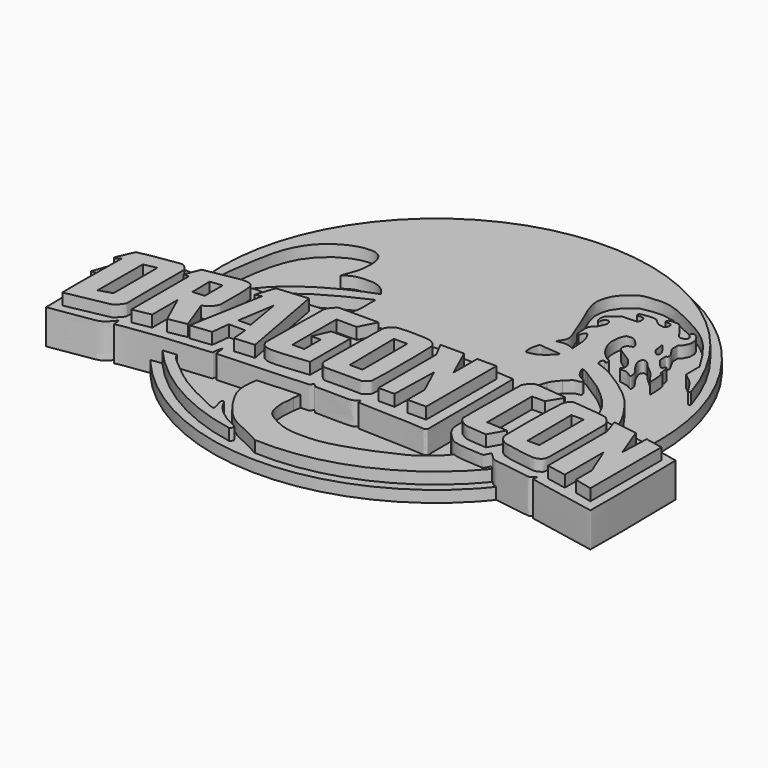
from build123d import *

# Parameters (mm, degrees)
F4_DEPTH = 6
F5_DEPTH = 9
F6_DEPTH = 12
F3_R     = 58.2680321176
F3_R_2   = 56.2680321176
F7_DEPTH = 3


with BuildPart() as f4:
    # F0 (on Top) → F4 (new body)
    with BuildSketch(Plane.XY):
        with BuildLine():
            ThreePointArc((50.2046270682, 32.5990865515), (-16.7313832275, 70.5566357957), (-58.0834932625, 5.662814714))
            add(Edge.make_bspline(
                [(-56.7946247756, 5.2932645194), (-56.9072491765, 5.3525443032), (-57.1453488244, 5.4763741354), (-57.5821193773, 5.672389242), (-57.9185015008, 5.6612390893), (-58.0834932625, 5.662814714)],
                knots=[0, 0, 0, 0, 0.3106893035, 0.6504797755, 1, 1, 1, 1], degree=3))
            add(Edge.make_bspline(
                [(-56.7946247756, 5.634940695), (-56.7946247756, 5.5210486365), (-56.7946247756, 5.407156578), (-56.7946247756, 5.2932645194)],
                knots=[0, 0, 0, 0, 0.3416761756, 0.3416761756, 0.3416761756, 0.3416761756], degree=3))
            add(Edge.make_bspline(
                [(-56.7946247756, 5.634940695), (-56.743940958, 7.2671798267), (-56.6456838315, 10.4314861922), (-56.7331520593, 14.5389266601), (-55.4633891473, 22.7353611724), (-54.1617687318, 29.6389256337), (-50.5897890483, 36.1168723343), (-44.7304711778, 39.9612863347), (-40.4860770295, 40.8741166974), (-37.6101297308, 40.5829749813), (-36.0593532544, 38.4827961794), (-35.7341565041, 35.7735493388), (-36.0278357089, 32.4009184257), (-36.969322235, 30.1083105362), (-37.420851473, 28.7852784917), (-37.6350395381, 28.1576830894)],
                knots=[0, 0, 0, 0, 0.0811415104, 0.1573032975, 0.2640365926, 0.3647803654, 0.4649779823, 0.5628837924, 0.6401346208, 0.7006202399, 0.7574588792, 0.8192083533, 0.8879467994, 0.946846281, 1, 1, 1, 1], degree=3))
            add(Edge.make_bspline(
                [(-37.6350395381, 28.1576830894), (-36.9020123713, 28.6742797134), (-35.3625484353, 29.7592079508), (-32.0226096017, 30.0311701045), (-28.9781587103, 29.8321241822), (-26.8192759482, 28.0309743743), (-26.3082476936, 27.1731155382), (-26.0944720358, 26.8142521381)],
                knots=[0, 0, 0, 0, 0.2057371384, 0.4320779901, 0.6506279419, 0.8538490957, 1, 1, 1, 1], degree=3))
            add(Edge.make_bspline(
                [(-50.9683191776, 7.4282060377), (-50.0897355561, 9.1461288779), (-48.1549941281, 12.9291910788), (-42.0082562909, 19.0156346462), (-32.7576914853, 24.3042127224), (-28.1550707663, 26.0380231586), (-26.0944720358, 26.8142521381)],
                knots=[0, 0, 0, 0, 0.2162082281, 0.4761151991, 0.7654561561, 1, 1, 1, 1], degree=3))
            add(Edge.make_bspline(
                [(-50.9683191776, 7.4282060377), (-50.5346785598, 7.504976032), (-49.5772579756, 7.674473929), (-48.2885622292, 7.7307833579), (-47.5835502148, 7.7615887858)],
                knots=[0, 0, 0, 0, 0.4529259397, 1, 1, 1, 1], degree=3))
            add(Edge.make_bspline(
                [(-25.3540985286, 24.1653900594), (-26.8552881088, 23.4932910546), (-30.1240573245, 22.0298273017), (-36.579939726, 18.4844991642), (-40.5144127202, 15.6900251466), (-44.4997206983, 12.1915121861), (-46.2658510708, 9.8325827108), (-47.1601372748, 8.4270560364), (-47.5835502148, 7.7615887858)],
                knots=[0, 0, 0, 0, 0.1794087162, 0.3906539828, 0.5668669146, 0.7447237719, 0.8791357199, 1, 1, 1, 1], degree=3))
            add(Edge.make_bspline(
                [(-27.7303513139, 12.6673979685), (-27.2486818484, 13.2179868784), (-26.3076778392, 14.2936339948), (-26.1352969689, 16.242044308), (-25.1319103155, 19.098439079), (-25.4017287693, 21.912956441), (-25.3693180923, 23.4456570399), (-25.3540985286, 24.1653900594)],
                knots=[0, 0, 0, 0, 0.186897327, 0.3651282604, 0.5890583856, 0.8070280333, 1, 1, 1, 1], degree=3))
            add(Edge.make_bspline(
                [(-27.7303513139, 12.6673979685), (-27.3267480987, 12.711642758), (-26.4365206138, 12.8092334765), (-24.8125175039, 11.887978411), (-23.3858019743, 10.910104507), (-22.5945804268, 10.3677995503)],
                knots=[0, 0, 0, 0, 0.2697704197, 0.5950325299, 1, 1, 1, 1], degree=3))
            add(Edge.make_bspline(
                [(-22.5945804268, 10.3677995503), (-22.4494425383, 10.1692900968), (-22.1047770931, 9.6978808054), (-20.541269939, 10.4450566992), (12.4683706928, 10.6003936274), (19.1899524017, 10.0772365955), (21.6048229486, 9.8892813548)],
                knots=[0, 0, 0, 0, 0.0748352198, 0.1777145488, 0.7045765412, 1, 1, 1, 1], degree=3))
            add(Edge.make_bspline(
                [(22.3375074565, 6.7731132731), (22.2050759519, 6.7121684444), (21.6804708525, 6.4707457707), (22.3820265231, 9.9005145642), (21.7795188996, 9.8918062997), (21.6048229486, 9.8892813548)],
                knots=[0, 0, 0, 0, 0.1934017225, 0.7661283481, 1, 1, 1, 1], degree=3))
            add(Edge.make_bspline(
                [(23.7141530961, 7.6335170306), (23.5129897112, 7.4387115421), (22.7964542586, 6.9261279039), (22.4677713883, 6.8165437695), (22.3375074565, 6.7731132731)],
                knots=[0.9396684612, 0.9396684612, 0.9396684612, 0.9396684612, 0.9760893428, 1, 1, 1, 1], degree=3))
            add(Edge.make_bspline(
                [(24.7681494802, 17.506653443), (24.5820762836, 17.0586454205), (24.2648384997, 16.2073215988), (24.1201965601, 15.3816965441), (23.6031723863, 14.5248965272), (23.0308114017, 14.1741195336), (23.3225715959, 13.8258667143), (23.6745692403, 13.8927180424), (24.073043796, 13.6874626518), (24.084510106, 13.1262821848), (23.9134607635, 12.3864586347), (23.2230506427, 12.1551260695), (23.0110411675, 11.3655136983), (23.9937166452, 11.3631300863), (24.1301903553, 9.8285262022), (24.1139508876, 8.5014299091), (23.9172018066, 7.9046271718), (23.8240178155, 7.7399094059), (23.7141530961, 7.6335170306)],
                knots=[0.4886615456, 0.4886615456, 0.4886615456, 0.4886615456, 0.5289439664, 0.5604071505, 0.5944543502, 0.6197125379, 0.6381612747, 0.6582483573, 0.6791704077, 0.7037719863, 0.7324620053, 0.760766481, 0.7860246628, 0.8136119764, 0.8536405418, 0.8942891369, 0.9197773168, 0.9396684612, 0.9396684612, 0.9396684612, 0.9396684612], degree=3))
            add(Edge.make_bspline(
                [(26.6395267099, 20.1954152435), (26.3304324892, 19.8599665702), (25.800711372, 19.1155739168), (25.2607428411, 18.6172505682), (24.9409139902, 17.9226181703), (24.7681494802, 17.506653443)],
                knots=[0.3822819269, 0.3822819269, 0.3822819269, 0.3822819269, 0.4220666272, 0.4512602819, 0.4886615456, 0.4886615456, 0.4886615456, 0.4886615456], degree=3))
            add(Edge.make_bspline(
                [(27.6289917529, 24.5619639754), (27.7723042031, 24.3496130639), (28.0047132596, 24.062317522), (28.8009821863, 23.4272012059), (29.636859997, 23.1896070116), (30.0117479679, 22.9145586663), (29.9724352086, 22.5030909475), (30.0837654817, 21.989256597), (29.0948646233, 21.9202442394), (28.3438289058, 21.8157880127), (27.506732088, 20.9669414955), (26.9301036432, 20.5107677809), (26.6395267099, 20.1954152435)],
                knots=[0.0901615916, 0.0901615916, 0.0901615916, 0.0901615916, 0.1174841509, 0.1513393374, 0.183460135, 0.2049406069, 0.2262289946, 0.2475173316, 0.2783858885, 0.308858332, 0.3448806575, 0.3822819269, 0.3822819269, 0.3822819269, 0.3822819269], degree=3))
            add(Edge.make_bspline(
                [(26.6180168837, 26.6914647073), (26.5538465905, 26.5589717891), (26.8569960314, 25.8120584593), (27.4068259364, 24.8911545906), (27.6289917529, 24.5619639754)],
                knots=[0.016726342, 0.016726342, 0.016726342, 0.016726342, 0.0478056157, 0.0901615916, 0.0901615916, 0.0901615916, 0.0901615916], degree=3))
            Line((26.6180168837, 26.6914647073), (27.4649984008, 26.4774558877))
            add(Edge.make_bspline(
                [(27.4649984008, 26.4774558877), (27.8447251207, 26.2618028632), (28.2272021191, 26.0392369144), (28.6180023104, 25.79575032)],
                knots=[0.0259787585, 0.0259787585, 0.0259787585, 0.0259787585, 0.0786197526, 0.0786197526, 0.0786197526, 0.0786197526], degree=3))
            add(Edge.make_bspline(
                [(28.6180023104, 25.79575032), (29.2730169015, 25.3876459339), (30.7542785317, 24.3682342053), (32.6443513786, 23.2826435246), (33.6572527885, 22.5470941514)],
                knots=[0.0786197526, 0.0786197526, 0.0786197526, 0.0786197526, 0.1668505672, 0.271269472, 0.271269472, 0.271269472, 0.271269472], degree=3))
            add(Edge.make_bspline(
                [(33.6572527885, 22.5470941514), (34.7273109728, 21.7700386363), (35.7844843208, 20.8287646233), (36.6501100361, 20.0402587652)],
                knots=[0.271269472, 0.271269472, 0.271269472, 0.271269472, 0.3815806064, 0.3815806064, 0.3815806064, 0.3815806064], degree=3))
            add(Edge.make_bspline(
                [(36.6501100361, 20.0402587652), (37.292958784, 19.4546823497), (38.2182681192, 18.5911826759), (38.9261192931, 17.7396287604), (40.1907067486, 16.2515716032), (40.6543056158, 15.204877891), (41.427662582, 13.675836954), (41.8512965291, 12.9822524326), (42.2321984163, 11.6714818261), (42.7690574845, 10.0860390174), (42.8662696975, 8.7455455769), (42.9171994328, 8.0432575196)],
                knots=[0.3815806064, 0.3815806064, 0.3815806064, 0.3815806064, 0.4635021268, 0.5226857979, 0.5987793491, 0.6611336223, 0.7325411021, 0.7835625135, 0.8470770152, 0.919883244, 1, 1, 1, 1], degree=3))
            add(Edge.make_bspline(
                [(42.9171994328, 8.0432575196), (42.9024112367, 7.8860698723), (42.8876230406, 7.7288822249), (42.9171994328, 7.6880422421)],
                knots=[0, 0, 0, 0, 0.1268041627, 0.1268041627, 0.1268041627, 0.1268041627], degree=3))
            add(Edge.make_bspline(
                [(42.9171994328, 7.6880422421), (42.9344599586, 7.6642083827), (43.1257206784, 7.7575143726), (45.8551757704, 7.4458161733), (48.3239047828, 7.1343355004), (48.3591927713, 7.0632003449), (48.360966146, 7.0652342401)],
                knots=[0.1268041627, 0.1268041627, 0.1268041627, 0.1268041627, 0.2008059711, 0.564047502, 0.89576174, 0.9238445121, 0.9238445121, 0.9238445121, 0.9238445121], degree=3))
            add(Edge.make_bspline(
                [(48.360966146, 7.0652342401), (48.3657752232, 7.0707498026), (48.3633706846, 7.1320535103), (48.360966146, 7.1933572181)],
                knots=[0.9238445121, 0.9238445121, 0.9238445121, 0.9238445121, 1, 1, 1, 1], degree=3))
            add(Edge.make_bspline(
                [(36.1157208681, 36.0662713647), (35.773357725, 36.4858516479), (35.204511851, 37.1829959455), (34.5882723775, 37.4692467297), (34.1907436738, 37.613005368), (33.7754735674, 37.5035723194), (33.5879262311, 37.122661341), (33.4619366475, 36.7760044404), (33.5151595421, 36.1514343553), (33.7044335309, 35.4511649474), (34.3396256687, 34.2498128459), (35.5498347865, 32.6712910878), (36.1843590789, 31.8617926362), (36.2593728387, 31.0428760427), (36.326071823, 30.2514060029), (35.6622035299, 30.6507695158), (34.6937180106, 31.2348511544), (34.0130033354, 31.48572503), (32.9441457606, 31.3654628006), (32.28324512, 31.6553200458), (32.6651787253, 32.0469486787), (32.8821835793, 32.4341376338), (32.9868619558, 32.860554244), (32.9094580545, 33.1418602913), (32.7310436474, 33.8484911551), (32.0263910281, 34.8534358437), (31.1432857657, 35.9342787069), (29.8649988477, 36.5882484781), (28.5359130178, 37.4984419519), (27.4601224946, 38.161771504), (27.000052561, 38.8707379421), (27.0444873894, 39.7725547848), (27.4931650602, 40.4061878694), (28.3634268271, 40.6775369894), (28.6861318691, 40.6918443679), (28.6875325403, 41.2436872028), (28.4581164465, 41.7714043897), (26.9722780992, 43.4134064283), (26.3111513175, 43.7394309182), (25.4630153224, 43.786860632), (24.6127119882, 43.6913954371), (24.3056166378, 43.2731313931), (23.7727135113, 42.0649496574), (23.6889356487, 40.7370872296), (23.6444567462, 38.952203693), (24.6178566036, 36.8141435024), (25.7908841259, 34.968695562), (27.1976592187, 33.7889357513), (27.8244944374, 33.2240920781), (28.5500194614, 33.1574458814), (28.8418247983, 32.3878141043), (28.7230648497, 31.9694577405), (28.2354771945, 31.7384956955), (28.0458532364, 32.4909892969), (27.2117936129, 31.9960839174), (27.4288521644, 30.6606168313), (28.009215765, 30.4642746618), (30.4548835525, 29.6660300862), (34.0195400483, 27.5927768021), (37.6116855637, 25.1111132301), (40.2664406582, 22.9959336235), (42.5594294472, 20.6619069218), (44.3947697855, 18.0705616128), (45.9872519944, 15.8908920919), (48.1726801168, 11.6889870771), (48.4515934779, 8.2272737019), (48.3841665129, 7.4580372127), (48.360966146, 7.1933572181)],
                knots=[0, 0, 0, 0, 0.0177520412, 0.0294955097, 0.0387661934, 0.0478175129, 0.0570219493, 0.0659034527, 0.0771853203, 0.0895299969, 0.1066794175, 0.1275480096, 0.1422274969, 0.1556889402, 0.1665379903, 0.1771264277, 0.1931301161, 0.2057182133, 0.2210383031, 0.2315453516, 0.2407247973, 0.250921016, 0.2602876483, 0.2679984619, 0.2801154945, 0.2964578956, 0.3137067922, 0.3312120086, 0.3499681451, 0.3663351398, 0.3793311095, 0.3926928694, 0.4054309766, 0.4191706672, 0.4265810759, 0.4361053434, 0.4477023269, 0.4692373412, 0.4820234701, 0.495313485, 0.508433687, 0.5185129293, 0.5349675916, 0.5520707142, 0.5713675926, 0.5937083873, 0.615708695, 0.6353392243, 0.648488793, 0.660214958, 0.6726524109, 0.6820721514, 0.6909277185, 0.7014679161, 0.7130802667, 0.7289451305, 0.7395794803, 0.7622060084, 0.7926790588, 0.8234277113, 0.8503709011, 0.8768088448, 0.9025287181, 0.9267600429, 0.9588644086, 0.9858460067, 1, 1, 1, 1], degree=3))
            add(Edge.make_bspline(
                [(16.6929047555, 37.9056371748), (16.5378166989, 37.8731615769), (16.1519920453, 37.792369499), (16.0214149151, 38.8807011871), (15.7006685701, 41.8815280031), (16.6900131774, 42.7208128146), (17.4043001531, 43.3402466116), (17.9470852188, 44.7398131588), (18.1407652765, 45.319563198), (18.0830024937, 45.7962846727), (17.9150820899, 46.2860621835), (17.6066163828, 46.6507546825), (17.1259829655, 46.604847688), (16.6794461622, 46.5499830364), (16.3072051755, 46.1938922326), (16.4480610932, 45.5658379064), (15.9890715373, 45.0477113275), (15.4814309005, 45.5655028786), (15.5446016032, 47.0262119797), (15.4989434034, 47.5635406429), (18.4280327463, 49.9285861052), (18.6026576542, 49.7817655266), (21.8157723772, 49.8735297856), (22.1440317332, 50.0382813448), (22.6565854809, 50.3880852006), (22.6407824068, 50.8765652436), (22.5840708013, 51.3513906128), (22.4512834387, 51.9202513812), (21.8559838386, 52.2416467245), (20.9063158813, 52.0696489057), (20.5473850596, 52.069665192), (20.3251862095, 52.44087076), (20.587738826, 53.0166087532), (21.7003942278, 53.1315613261), (23.3117089717, 53.4189694152), (24.656699149, 53.2679853616), (25.345266583, 52.635049732), (26.1319237527, 51.8334616635), (27.3503460973, 51.4742092473), (28.2556834883, 51.5465995508), (28.6617406688, 52.2458890516), (28.6223427788, 53.1554203659), (28.0444791752, 53.5615430537), (27.0224589264, 53.3436600317), (26.7002655144, 53.6254959194), (26.7733073997, 54.0183060439), (27.0496150095, 54.3814046425), (27.7756922212, 54.59319388), (29.1701202191, 54.4445387012), (29.949175178, 54.5530942808), (32.7518683822, 50.5542217843), (33.1951742042, 49.969337053), (33.7662590367, 49.8746249102), (34.0790851541, 49.9074089827), (34.4946728832, 49.9830810986), (34.7922244192, 50.2536587571), (35.1257770617, 50.5620322235), (35.0696743785, 51.0029187727), (35.077925207, 51.4712460707), (34.6007750321, 51.6211318048), (34.3438143712, 51.9747067321), (34.2736995383, 52.3186333719), (34.2915507816, 52.7803302136), (34.8733527983, 52.9464246023), (35.4230048824, 52.680435122), (36.0566369917, 52.1347706721), (36.3007034078, 51.5836726817), (36.8546541663, 50.9852926894), (36.8800545821, 48.9921454267), (36.4631679072, 48.3780509903), (36.1806478572, 47.6030393539), (35.3211527806, 47.0155596986), (35.3439526085, 46.736657981), (35.3967328653, 46.2282165886), (35.2217950277, 45.1414556019), (35.8265095235, 44.1835865704), (36.8473395961, 42.7795710718), (36.9400870955, 42.4319879297), (36.9579347946, 41.6836715779), (36.4960662835, 41.6710121171), (36.4920712765, 41.282369265), (36.4078239677, 40.9174032015), (36.5189597314, 40.3650052747), (36.4062662281, 39.8246083602), (36.7886427258, 39.2559671695), (37.3673789538, 38.6569195227), (38.0564323159, 37.77587332), (38.4851959995, 37.274307465), (38.716037707, 37.1595630801), (39.0828724458, 37.1884641788), (39.173013311, 37.3592233278), (39.1976255109, 37.5964670077), (39.239344905, 37.7366151786), (39.5582998617, 38.0031728314), (39.8421003504, 37.6958445452), (39.9083644975, 37.226573246), (40.186994638, 35.9887401404), (40.2044754575, 34.7634139251), (40.7532527796, 36.4286755287), (41.117968664, 30.9302802653), (40.7409797268, 30.9299735407), (38.9824606101, 33.6647336712), (37.5516217359, 34.8908932322), (36.1487326538, 36.0131769065), (36.0881901491, 36.0706836304), (36.104094763, 36.0638901476), (36.1157208681, 36.0662713647)],
                knots=[0, 0, 0, 0, 0.0072579471, 0.0180561611, 0.0376323485, 0.0497612202, 0.0607287624, 0.0744298809, 0.0832556883, 0.0908187432, 0.098965474, 0.1063767916, 0.1139281961, 0.121514272, 0.12897354, 0.1378090834, 0.1458158546, 0.1539345463, 0.1672217069, 0.1762705342, 0.1971821312, 0.2040560336, 0.2237035484, 0.2314352325, 0.2395601814, 0.2471425349, 0.2550562655, 0.2633508278, 0.2722249975, 0.283267886, 0.28972942, 0.2963640507, 0.3043445698, 0.3159104701, 0.3307104076, 0.3435471863, 0.3541724037, 0.3660703986, 0.3787390865, 0.3889729032, 0.3985618536, 0.4088791041, 0.4177267616, 0.4289907123, 0.4355074375, 0.4421649073, 0.4494710732, 0.4591794303, 0.4722550993, 0.4821277725, 0.5065671766, 0.5166961916, 0.524502932, 0.5309457458, 0.5380782022, 0.5452744696, 0.5525806355, 0.5599587921, 0.5672259673, 0.5747103116, 0.5820164775, 0.58874109, 0.5958316026, 0.6037722511, 0.6125980584, 0.6228209221, 0.6313814476, 0.6414238749, 0.6569458396, 0.6667032927, 0.676919875, 0.6879962177, 0.6933766826, 0.7012632179, 0.7127558399, 0.7251193843, 0.7396993758, 0.7468821122, 0.7557346169, 0.7621961509, 0.7685362575, 0.7755696607, 0.7839424139, 0.7921474212, 0.8010903422, 0.8115831545, 0.8237159293, 0.8326961132, 0.8382895729, 0.8447511069, 0.8494706529, 0.8548511178, 0.859291796, 0.8658139798, 0.8721215648, 0.8798056671, 0.893460283, 0.9030492333, 0.9101018274, 0.9338611558, 0.9375953062, 0.9570651707, 0.9747596003, 0.9887931695, 0.9907067635, 0.9923158978, 0.9923158978, 0.9923158978, 0.9923158978], degree=3))
            add(Edge.make_bspline(
                [(16.6929047555, 37.9056371748), (16.7445179414, 38.1581894685), (16.8404975069, 38.6278341714), (17.006259837, 39.1837817639), (17.2805199877, 39.3835604153), (17.5034212038, 39.4441484336), (17.8224980713, 39.3836106257), (18.0209448852, 39.0057353), (18.424880537, 38.2985744824), (18.7292817613, 37.7417817361), (18.7965439146, 37.4746491999), (18.8500494569, 37.0448065253), (19.2440747223, 36.289598469), (19.1691515815, 33.1683640044), (19.5026279255, 32.534789516), (19.2250664994, 32.5783658883), (19.1047992557, 32.5972475111)],
                knots=[0, 0, 0, 0, 0.0821824876, 0.1528260521, 0.2051712283, 0.2497832217, 0.2997614285, 0.3595323571, 0.4465038087, 0.5214242788, 0.5698262789, 0.6271126795, 0.7156916141, 0.8841676151, 0.9498098787, 1, 1, 1, 1], degree=3))
            add(Edge.make_bspline(
                [(19.1047992557, 32.5972475111), (18.5200764199, 32.8700466934), (17.2650896814, 33.4555537662), (15.6162022347, 33.0959295328), (14.7355636582, 32.9038612545)],
                knots=[0, 0, 0, 0, 0.4659195336, 1, 1, 1, 1], degree=3))
            add(Edge.make_bspline(
                [(44.6303412318, 42.4088686705), (44.1678474829, 43.1966171864), (43.0694272366, 45.0675158116), (39.802507905, 49.8588232199), (35.9946406885, 53.6035988977), (29.9903461685, 56.9341887131), (24.4850984043, 59.5121959931), (21.245362122, 60.0817167923), (18.5670597248, 59.8821645789), (15.5329183907, 59.5554983296), (14.0303491199, 58.2219182547), (12.4277937806, 56.9665231178), (11.0920554256, 55.0524875349), (10.6067838751, 53.3041393086), (9.9782854336, 50.8404385363), (12.1301464689, 45.4962770556), (13.396663567, 42.9661906388), (14.7014680552, 39.0336991696), (15.674883335, 37.3368402605), (16.1842179598, 34.9624620057), (15.2623918598, 33.8789008535), (14.9054833116, 33.2183440218), (14.7355636582, 32.9038612545)],
                knots=[0, 0, 0, 0, 0.0493909807, 0.1173033221, 0.183712457, 0.2586166023, 0.3289345081, 0.3794238768, 0.4260653594, 0.4749385395, 0.5145142368, 0.5551136811, 0.5980728397, 0.6357087926, 0.680272285, 0.747244533, 0.797899775, 0.8541894576, 0.8954395328, 0.9375444066, 0.9702656805, 1, 1, 1, 1], degree=3))
            add(Edge.make_bspline(
                [(44.6303412318, 42.4088686705), (44.6303412318, 41.9931596437), (44.6303412318, 40.9587410276), (44.6303412318, 39.0841893554), (44.6303412318, 37.9629768431)],
                knots=[0, 0, 0, 0, 0.4018769773, 1, 1, 1, 1], degree=3))
            add(Edge.make_bspline(
                [(49.5361499488, 32.520595938), (49.2262577264, 32.9671743414), (48.5909578932, 33.88269001), (47.696043062, 35.5155596569), (46.3169466393, 36.6813128581), (45.2086713889, 37.5234994583), (44.6303412318, 37.9629768431)],
                knots=[0, 0, 0, 0, 0.2368241254, 0.4855053352, 0.7315217676, 1, 1, 1, 1], degree=3))
            add(Edge.make_bspline(
                [(49.5361499488, 32.520595938), (49.6329811674, 32.421646566), (49.8354469262, 32.2021217726), (50.0934716697, 32.4668306113), (50.2046270682, 32.5990865515)],
                knots=[0, 0, 0, 0, 0.4683659655, 1, 1, 1, 1], degree=3))
        make_face()
        with BuildLine():
            add(Edge.make_bspline(
                [(13.2672535256, 29.4605158269), (13.0546831305, 29.3310557006), (12.9780582435, 28.7099731048), (12.6580662521, 27.8861255101), (12.6154662684, 26.895476162), (12.6107612572, 26.1152601993), (12.8455246818, 25.357837324), (13.0540169321, 25.3463005652), (13.5809959371, 25.4370725187), (14.9335143268, 25.6561843541), (16.5155050279, 26.4804916173), (18.9078927637, 28.6363059367), (18.7958025036, 29.1498853304), (16.3526261571, 29.2663748691), (14.8807356515, 29.3475074675), (13.5588098559, 29.638080155), (13.2672535256, 29.4605158269)],
                knots=[0, 0, 0, 0, 0.0604685275, 0.1266229913, 0.1942931768, 0.2577091891, 0.3152891343, 0.3419484798, 0.3903161403, 0.4686015811, 0.5670239016, 0.6870205459, 0.7215005707, 0.8239078677, 0.9170628536, 1, 1, 1, 1], degree=3))
        make_face(mode=Mode.SUBTRACT)
        with BuildLine():
            add(Edge.make_bspline(
                [(32.7647812665, 44.9209474027), (32.8418197159, 45.0480984598), (33.4948228289, 44.0612702026), (34.3391901492, 43.2584616553), (34.8468728337, 42.2176989183), (34.7870670441, 42.1267845787), (34.864633785, 41.2946697526), (34.6657133042, 41.2417092032), (34.4063726303, 41.236219855), (34.0957605607, 41.1712991671), (32.9079061226, 42.7455098508), (33.1166666685, 42.8098522502), (32.6497834877, 44.7311449181), (32.7647812665, 44.9209474027)],
                knots=[0, 0, 0, 0, 0.1051427454, 0.241032552, 0.350193187, 0.389451954, 0.4856292942, 0.5291499201, 0.5827293142, 0.6429891292, 0.7894706055, 0.843050032, 1, 1, 1, 1], degree=3))
        make_face(mode=Mode.SUBTRACT)
    extrude(amount=F4_DEPTH)


with BuildPart() as f4b:
    # F0 (on Top) → F4, piece 2 (new body)
    with BuildSketch(Plane.XY):
        with BuildLine():
            ThreePointArc((-5.9422926341, -39.4621712035), (19.3133198421, -34.7703489333), (39.7998097434, -19.2731592109))
            add(Edge.make_bspline(
                [(29.6710466946, -19.0613246448), (29.9889896662, -19.2079401263), (30.9113480955, -19.5505704592), (33.2415521979, -19.781250181), (34.7737928201, -19.8415350469), (38.0468342315, -20.0814423489), (38.1322334227, -19.9695396325), (38.8903846796, -18.5850903432), (39.0777604856, -18.44631315), (39.5009952091, -18.9295370278), (39.7998097434, -19.2731592109)],
                knots=[0.7387932181, 0.7387932181, 0.7387932181, 0.7387932181, 0.7662243898, 0.8128495832, 0.8547967332, 0.9069469463, 0.9194267569, 0.9568912879, 0.9689731011, 1, 1, 1, 1], degree=3))
            add(Edge.make_bspline(
                [(28.2211229205, -20.8663698286), (28.5532039615, -20.5184044992), (29.1599192779, -19.8811931098), (29.510875969, -19.3192821088), (29.6710466946, -19.0613246448)],
                knots=[0, 0, 0, 0, 0.5465278871, 1, 1, 1, 1], degree=3))
            add(Edge.make_bspline(
                [(19.9911892414, -26.365051046), (20.8491396487, -26.0284577554), (22.7006630254, -25.302063385), (25.796632924, -22.9442962221), (27.4383408521, -21.5372587672), (28.2211229205, -20.8663698286)],
                knots=[0, 0, 0, 0, 0.311188031, 0.671567854, 1, 1, 1, 1], degree=3))
            add(Edge.make_bspline(
                [(-11.4223649725, -20.0674962252), (-11.4129834546, -20.5820060274), (-11.3945704528, -21.591828749), (-11.7521791553, -23.0319968234), (-11.6217655774, -23.9730446595), (-11.5609575749, -25.2833589863), (-11.2884304913, -26.3576836599), (-11.137137615, -27.0368382517), (-10.9771219191, -27.3630713888), (-10.6115532431, -28.037059456), (-10.0408500964, -28.6090186688), (-9.3205214922, -29.1603603088), (-8.257848686, -29.8091113069), (-6.8114921503, -30.6046029523), (-5.0668095347, -31.29394068), (-3.0366562679, -31.8222989793), (-0.1381429295, -32.0085400813), (4.0051304922, -31.9054032195), (7.4956178903, -31.1158845758), (10.45895331, -30.2077259849), (15.540878546, -28.4919059744), (18.5211522752, -27.0675987063), (19.9911892414, -26.365051046)],
                knots=[0, 0, 0, 0, 0.0463242852, 0.0909201644, 0.1271452392, 0.169627141, 0.2094651309, 0.239554643, 0.2617692473, 0.2937470175, 0.3274267444, 0.3625365423, 0.403891386, 0.4518237524, 0.5026829074, 0.5559523385, 0.6193537398, 0.6956275381, 0.7654767175, 0.8309607843, 0.9166204455, 1, 1, 1, 1], degree=3))
            add(Edge.make_bspline(
                [(-11.4223649725, -20.0674962252), (-11.3295242611, -19.4083497633), (-11.2364883158, -18.7521844109), (-11.1436476043, -18.093037949)],
                knots=[0, 0, 0, 0, 1.9940333136, 1.9940333136, 1.9940333136, 1.9940333136], degree=3))
            add(Edge.make_bspline(
                [(-11.1436476043, -18.093037949), (-13.7140060899, -18.2613716336), (-18.0371433408, -18.4802652718), (-22.1086186539, -18.6719495981)],
                knots=[0.648925281, 0.648925281, 0.648925281, 0.648925281, 0.6983544843, 0.6983544843, 0.6983544843, 0.6983544843], degree=3))
            add(Edge.make_bspline(
                [(-22.3164577037, -20.3040745109), (-22.2472340209, -19.758843394), (-22.1778423367, -19.217180715), (-22.1086186539, -18.6719495981)],
                knots=[0, 0, 0, 0, 1.6453050786, 1.6453050786, 1.6453050786, 1.6453050786], degree=3))
            add(Edge.make_bspline(
                [(-22.3164577037, -20.3040745109), (-22.4104644896, -21.3698193426), (-22.599094178, -23.5083669689), (-21.5267610859, -26.5377382196), (-19.6392126505, -29.6235306665), (-17.8261543567, -32.0630082297), (-16.0724331909, -33.9904729669), (-13.5694061347, -35.8916501611), (-9.1991803939, -37.5932081689), (-7.0195723242, -39.0104931821), (-5.9422926341, -39.4621712035)],
                knots=[0, 0, 0, 0, 0.1213004835, 0.2424832038, 0.3724918995, 0.4913667503, 0.5997130639, 0.7199297645, 0.8678313386, 1, 1, 1, 1], degree=3))
        make_face()
    extrude(amount=F4_DEPTH)


with BuildPart() as f4c:
    # F0 (on Top) → F4, piece 3 (new body)
    with BuildSketch(Plane.XY):
        with BuildLine():
            add(Edge.make_bspline(
                [(-41.8352228593, -19.9243533115), (-43.0312733259, -20.0494568329), (-44.223837241, -20.1767656719), (-45.4164011561, -20.3040745109)],
                knots=[0.9648730132, 0.9648730132, 0.9648730132, 0.9648730132, 1, 1, 1, 1], degree=3))
            ThreePointArc((-45.4164011561, -20.3040745109), (-30.9307344607, -32.1851190967), (-13.331754607, -38.6092663682))
            add(Edge.make_bspline(
                [(-17.0426741242, -35.1028442383), (-16.5863003245, -35.4461059495), (-15.6109924711, -36.1820574701), (-13.7838266009, -36.8131587571), (-12.8779420291, -37.4176334374), (-12.6811475631, -37.8777630901), (-13.0839631615, -38.4300546348), (-13.331754607, -38.6092663682)],
                knots=[0, 0, 0, 0, 0.2505838761, 0.5131913973, 0.7020587984, 0.8203230684, 1, 1, 1, 1], degree=3))
            add(Edge.make_bspline(
                [(-40.2302891016, -22.1484415233), (-39.5538325651, -22.7453334697), (-38.1575824108, -23.9773571507), (-35.7332956974, -25.9527539286), (-32.8797930055, -28.0251826358), (-29.2946349564, -30.160127584), (-24.9114809276, -32.1900660172), (-22.9029549086, -33.1772071078), (-21.5073135856, -33.8400227363), (-21.2524581608, -33.4957291133), (-21.3342515642, -33.1584281776), (-21.5160193189, -32.7084097026), (-21.6483743955, -31.7135157531), (-21.8618751424, -31.4635497295), (-22.1021911388, -30.110287794), (-21.5151071201, -30.1136894317), (-21.1202458867, -30.5002731883), (-20.7967126463, -31.4098738882), (-19.9750736277, -32.4546056087), (-18.9113862967, -33.7281310863), (-17.7006981221, -34.61877063), (-17.0426741242, -35.1028442383)],
                knots=[0, 0, 0, 0, 0.0720992696, 0.1488175676, 0.2301156926, 0.3205012091, 0.4160291849, 0.4832176591, 0.5327865385, 0.5554461015, 0.5796415476, 0.6110683746, 0.6532600368, 0.6812254472, 0.7279504925, 0.7538244075, 0.7850799306, 0.8273416257, 0.8773272617, 0.9333258494, 1, 1, 1, 1], degree=3))
            add(Edge.make_bspline(
                [(-40.2302891016, -22.1484415233), (-40.6241250746, -21.7954814734), (-41.3762826929, -21.124199428), (-41.6871488493, -20.3079889918), (-41.8352228593, -19.9243533115)],
                knots=[0, 0, 0, 0, 0.5249873353, 1, 1, 1, 1], degree=3))
        make_face()
    extrude(amount=F4_DEPTH)


with BuildPart() as f5:
    # F1 (on Top) → F5 (new body)
    with BuildSketch(Plane.XY):
        with BuildLine():
            add(Edge.make_bspline(
                [(-59.6398003399, 5.7134046219), (-59.5297687978, 5.714448729), (-59.5450051083, 5.6235197668), (-58.4025444324, 5.7033602147), (-57.6480493484, 5.6098081624), (-56.9171877742, 5.3160282089), (-56.6279605335, 5.1084389413), (-56.3814523621, 5.0509240949), (-56.1126046595, 6.2471025787), (-55.8958021549, 6.3643009138), (-50.5234663581, 7.4775752035), (-47.912467701, 7.6362296465), (-43.3566601089, 8.0953263882), (-42.1621995654, 7.9450271438), (-41.2695118071, 7.7045039222), (-40.0221182573, 6.342189231), (-39.9227572833, 6.3527666687), (-38.8926522397, 8.7568743518), (-39.1081674118, 8.755403561), (-26.3356454582, 10.2068608748), (-27.1162218365, 9.7008207034), (-26.8724693489, 9.760765242), (-27.0791101887, 9.4753795378), (-26.4991000066, 6.653981206), (-26.2379168756, 6.6292157152), (-25.6810553206, 7.6045859272), (-25.2231383649, 8.4560106401), (-24.3146964616, 9.1698327112), (-23.3646949285, 9.8446104437), (-22.2383631771, 10.2335299382), (-20.3261137955, 10.3951154192), (-5.7810651357, 10.7667810832), (2.8474857785, 10.8351422671), (15.4814272655, 10.4977174374), (21.7800247382, 9.8858360351), (22.2107925399, 10.0271779344), (22.0156768023, -18.0093357225), (22.2086448235, -18.215730441), (21.9798894816, -18.3950545368), (21.3836977867, -18.674839277), (21.2402959076, -18.3826021751), (3.9028532137, -17.8762080496), (3.6715121086, -17.8239262783), (3.7028698633, -16.7077101664), (3.470739766, -17.0247873724), (3.0464238283, -17.2968048711), (2.5389196306, -17.6436924683), (1.743146579, -18.2502472699), (-7.3843561702, -17.748031502), (-7.4723804427, -17.9848334597), (-8.1946188727, -17.0877470355), (-8.389564485, -17.0881884922), (-8.8815012669, -17.9596917744), (-8.9181293943, -17.9174434625), (-32.2127497464, -19.2600432521), (-32.253717503, -19.1467908349), (-32.4717337056, -19.010323491), (-32.5441572198, -16.4217109826), (-32.7994533168, -16.4147008876), (-33.3700120745, -19.0887319887), (-32.7324143486, -19.3057616256), (-45.7467367392, -20.0973635653), (-56.3882200127, -21.7997542456), (-56.7037176264, -22.1150730117), (-56.8240705651, -19.9346520562), (-57.2168787568, -20.4812881566), (-58.0576502544, -21.4793412294), (-59.4162556471, -23.0283486588), (-65.5180277535, -23.6914187699), (-72.0829179196, -24.8171772178), (-72.3085308032, -24.8230542659), (-72.4227471327, -6.6063450765), (-71.9985304292, -6.2714541627), (-75.051558764, -6.8342597746), (-74.7907247366, -6.5404206288), (-71.4093387069, 3.4111246717), (-71.6358388209, 3.3186375347), (-60.570768137, 5.7045705181), (-59.6398003399, 5.7134046219)],
                knots=[0, 0, 0, 0, 0.0038058591, 0.0131516798, 0.0219547664, 0.0301124822, 0.0356129397, 0.039255335, 0.0490311319, 0.0539331891, 0.0748985847, 0.092241827, 0.1116874246, 0.1217229401, 0.1309932588, 0.1432527873, 0.1454832305, 0.1603868761, 0.1629705413, 0.1953759385, 0.1980287046, 0.2011009778, 0.2054465255, 0.2213156642, 0.2244699872, 0.2339520682, 0.2436168513, 0.2535229192, 0.2636924359, 0.2732876894, 0.2858614211, 0.3207846004, 0.3504392092, 0.3843602258, 0.4062573701, 0.4102039791, 0.4595746849, 0.4648992951, 0.4693989587, 0.4763936597, 0.4826127678, 0.5213871908, 0.526423879, 0.5349770398, 0.5387980427, 0.5457106567, 0.5525378971, 0.5625319266, 0.5904501127, 0.5944108551, 0.6039069824, 0.6075699247, 0.6161712336, 0.6218123783, 0.6668167429, 0.6697411017, 0.6738969942, 0.6888261289, 0.6910692548, 0.7063644469, 0.7096218033, 0.7426105367, 0.7739694903, 0.7768653535, 0.7893156474, 0.7939921169, 0.8047415522, 0.8174246435, 0.841634943, 0.8650535874, 0.8681339492, 0.9081194009, 0.9122556959, 0.9277639513, 0.9309366622, 0.9609460035, 0.9677989405, 1, 1, 1, 1], degree=3))
        make_face()
    extrude(amount=F5_DEPTH)


with BuildPart() as f5b:
    # F1 (on Top) → F5, piece 2 (new body)
    with BuildSketch(Plane.XY):
        with BuildLine():
            add(Edge.make_bspline(
                [(52.6984557509, -22.0666453242), (61.1466039143, -23.7474300651), (70.2058296609, -25.5497905474), (70.6920502039, -25.4711061741), (70.4792904861, -11.0712107371), (70.2781900764, 2.5395653211)],
                knots=[0, 0, 0, 0, 0.431047172, 0.4622259888, 1, 1, 1, 1], degree=3))
            add(Edge.make_bspline(
                [(70.2781900764, 2.5395653211), (65.8706158151, 3.4590317378), (57.7045865224, 5.0176356887), (48.3908776562, 7.3520780854), (40.7337889827, 7.8719452386), (31.0839032792, 9.1276378874), (29.1693554554, 8.9648088752), (28.0306327122, 8.1437850493), (26.3807387685, 6.4030979136), (25.4513053784, 4.8811084994), (25.5750159826, -14.5513802488), (26.090259512, -14.9432068231), (26.6467244033, -16.4616820516), (28.7719236408, -18.2811177185), (29.6182907075, -19.4546236254), (35.4754745995, -20.0447364164), (38.0979267464, -20.0498337783), (38.2197403385, -20.0041259828), (38.9817212653, -18.2832267601), (39.1869723572, -18.5613326995), (39.9745090872, -19.2941214885), (40.960853671, -20.2320805509), (41.8150096328, -20.5187892555), (51.2005648801, -21.7501191345), (51.5272873214, -21.8248899284), (52.9202060821, -20.8023613121), (52.7132364939, -21.0666108235), (52.7049257292, -21.6288999756), (52.6984557509, -22.0666453242)],
                knots=[0, 0, 0, 0, 0.0843118478, 0.1554712879, 0.2223765337, 0.2940858063, 0.3246715336, 0.351380721, 0.3852919074, 0.4206204244, 0.5218330932, 0.5411711564, 0.5689904082, 0.6076561703, 0.6355939187, 0.6925174126, 0.728793309, 0.7373904304, 0.7678222591, 0.7767444583, 0.8011552217, 0.8274446146, 0.8523791027, 0.9228860506, 0.9421786835, 0.969117117, 0.9759540903, 1, 1, 1, 1], degree=3))
        make_face()
    extrude(amount=F5_DEPTH)


with BuildPart() as f6:
    # F2 (on Top) → F6 (new body)
    with BuildSketch(Plane.XY):
        with BuildLine():
            add(Edge.make_bspline(
                [(-71.3236555457, -3.6705303937), (-71.6987163123, -3.2607210005), (-69.3255903195, 1.0417709253), (-69.8039469837, 1.1175708043), (-58.4726586921, 3.290744722), (-58.4385576208, 2.6640394561), (-58.0720843759, 2.6265042947), (-57.537753744, 2.0803060207), (-56.8049104764, 1.295530717), (-57.107932026, 0.2043598982), (-56.7220581312, -17.5843930628), (-56.8902223208, -17.8305564145), (-57.4406773604, -18.6783296867), (-57.960646359, -19.2890291821), (-58.9374618201, -20.0228997818), (-59.3723876315, -19.9711024276), (-70.0235818316, -22.1717333491), (-70.0809834043, -22.0985558532), (-70.1363301413, -3.3780544369), (-69.8590303308, -2.8364782313), (-71.1177705122, -3.895490262), (-71.3236555457, -3.6705303937)],
                knots=[0, 0, 0, 0, 0.0795441755, 0.0896166601, 0.2070821301, 0.2278197133, 0.2463993927, 0.277660842, 0.3110817916, 0.3530307889, 0.5014168436, 0.5250883793, 0.5580325508, 0.5920689417, 0.6278798269, 0.6593004689, 0.7745946344, 0.7880630356, 0.9423647951, 0.956335195, 1, 1, 1, 1], degree=3))
        make_face()
        Polygon((-65.0384351611, -16.8952848762), (-64.9711191654, -2.2349301726), (-61.7062747478, -1.56089128), (-61.7062747478, -15.8842261881), align=None, mode=Mode.SUBTRACT)
    extrude(amount=F6_DEPTH)


with BuildPart() as f6b:
    # F2 (on Top) → F6, piece 2 (new body)
    with BuildSketch(Plane.XY):
        with BuildLine():
            Line((-18.354780972, -5.5386195891), (-15.9353613853, -5.5001662113))
            Line((-15.9353613853, -5.5001662113), (-15.9353613853, -10.8451852575))
            Line((-15.9353613853, -10.8451852575), (-19.0076399595, -10.8451852575))
            Line((-19.0076399595, -10.8451852575), (-19.0076399595, 3.4594710451))
            Line((-19.0076399595, 3.4594710451), (-13.7079600245, 3.4594710451))
            Line((-13.7079600245, 3.4594710451), (-11.4778349512, 7.7995401807))
            add(Edge.make_bspline(
                [(-11.4778349512, 7.7995401807), (-15.8725510299, 7.7525327463), (-21.1491956225, 7.7124241626), (-21.7476089904, 7.8651635528), (-22.3886995138, 7.4034810792), (-23.2621102296, 6.4794399744), (-23.8481503712, 5.3913848926), (-23.6556039847, 5.3539352664), (-24.2106678791, -13.6794650266), (-23.8307708168, -13.7035649222), (-23.4021492622, -14.7266276459), (-22.3445293221, -15.1069381402), (-20.8156791958, -15.5557508053), (-15.410373556, -14.9077056856), (-11.4805577323, -14.53573443)],
                knots=[0, 0, 0, 0, 0.168857193, 0.2041735349, 0.2482656958, 0.3122776741, 0.3674876742, 0.395994708, 0.6278112997, 0.6636546914, 0.7151126956, 0.7698542899, 0.8332571505, 1, 1, 1, 1], degree=3))
            Line((-11.4805577323, -14.53573443), (-11.4805577323, -1.3472014107))
            Line((-11.4805577323, -1.3472014107), (-16.5114142001, -1.3472014107))
            Line((-16.5114142001, -1.3472014107), (-18.354780972, -5.5386195891))
        make_face()
    extrude(amount=F6_DEPTH)


with BuildPart() as f6c:
    # F2 (on Top) → F6, piece 3 (new body)
    with BuildSketch(Plane.XY):
        Polygon((6.5926047973, -14.7974230349), (10.77248808, -14.7974230349), (11.1144790426, -2.3175752722), (14.4583852962, -9.5848031342), (14.4583852962, -15.1779064909), (19.3222481757, -15.1779064909), (19.3222481757, 7.7652288601), (14.3063887954, 7.7652288601), (14.3063887954, 0), (10.7344882563, 7.9554701224), (4.5406618156, 7.9554701224), (6.5926047973, 4.0747271851), align=None)
    extrude(amount=F6_DEPTH)


with BuildPart() as f6d:
    # F2 (on Top) → F6, piece 4 (new body)
    with BuildSketch(Plane.XY):
        with BuildLine():
            Line((36.7433167994, 1.812472241), (38.8651378453, 5.3383680061))
            add(Edge.make_bspline(
                [(38.8651378453, 5.3383680061), (38.8820564796, 5.4978399912), (38.9170910249, 5.8275664191), (38.3427588416, 5.6809481927), (30.6532410326, 6.7662987268), (30.2146948778, 6.2597386458), (29.5285509806, 5.8864983719), (28.4321290522, 4.4803990283), (28.679702018, 3.1772187512), (28.0696065134, -14.2101405127), (28.3567902883, -14.3449502173), (28.5571874467, -15.0518231806), (29.0504014752, -15.4791807814), (29.5955743746, -15.9711916418), (30.7462882469, -16.5930155509), (32.0161650867, -16.8487668176), (34.722568802, -16.9293956187), (36.4724472165, -17.1279162169)],
                knots=[0, 0, 0, 0, 0.0315466637, 0.0653464746, 0.2054191052, 0.2456197355, 0.2882170899, 0.34967501, 0.4190276979, 0.6266123491, 0.6552663078, 0.6951636024, 0.7360997699, 0.779497278, 0.8354000896, 0.8922180555, 1, 1, 1, 1], degree=3))
            Line((36.4724472165, -17.1279162169), (38.7748479843, -13.1047777832))
            Line((38.7748479843, -13.1047777832), (33.3574339747, -12.7883506939))
            Line((33.3574339747, -12.7883506939), (33.3574339747, 1.812472241))
            Line((33.3574339747, 1.812472241), (36.7433167994, 1.812472241))
        make_face()
    extrude(amount=F6_DEPTH)


with BuildPart() as f6e:
    # F2 (on Top) → F6, piece 5 (new body)
    with BuildSketch(Plane.XY):
        Polygon((59.9199309945, 2.4815041106), (53.5766333342, 3.4472357947), (54.9838989973, -0.8305818774), (54.9838989973, -19.9712812901), (60.1588338614, -20.9770034999), (60.1588338614, -8.2742860541), (63.2956027985, -16.0754397511), (63.2956027985, -21.2903469801), (67.9696127772, -22.4046520889), (67.9696127772, 0.77290216), (63.4068921208, 1.7014902551), (63.1101280451, -5.8386432938), align=None)
    extrude(amount=F6_DEPTH)


with BuildPart() as f6f:
    # F2 (on Top) → F6, piece 6 (new body)
    with BuildSketch(Plane.XY):
        Polygon((-29.1561651975, 7.200315129), (-37.209128324, 6.4734742045), (-38.8611517847, 1.5610851115), (-37.252034992, 1.9638875965), (-40.7216958702, -17.2699131072), (-35.3412106633, -16.6657101363), (-34.7880758345, -11.9109310396), (-30.4815535727, -11.9109310396), (-30.1618631929, -16.0615071654), (-24.9322317541, -15.658704564), align=None)
        Polygon((-34.330625087, -9.3455044553), (-32.7944867313, 0.3447470954), (-31.1431363225, -9.3455044553), align=None, mode=Mode.SUBTRACT)
    extrude(amount=F6_DEPTH)


with BuildPart() as f6g:
    # F2 (on Top) → F6, piece 7 (new body)
    with BuildSketch(Plane.XY):
        with BuildLine():
            Line((-45.0987257063, 5.0730230287), (-54.1340522468, 3.4472357947))
            Line((-54.1340522468, 3.4472357947), (-55.7713247836, -0.5130867939))
            Line((-55.7713247836, -0.5130867939), (-54.3766133487, -0.5130867939))
            Line((-54.3766133487, -0.5130867939), (-54.3766133487, -19.2144103348))
            Line((-54.3766133487, -19.2144103348), (-49.6401377939, -18.3391953095))
            Line((-49.6401377939, -18.3391953095), (-49.6401377939, -10.0459046662))
            Line((-49.6401377939, -10.0459046662), (-46.0689626634, -17.9393216968))
            Line((-46.0689626634, -17.9393216968), (-41.3650345005, -17.0701208408))
            Line((-41.3650345005, -17.0701208408), (-44.3710461259, -8.9529706165))
            add(Edge.make_bspline(
                [(-45.0987257063, 5.0730230287), (-44.5806395685, 5.1149064162), (-43.5891120153, 5.1950639995), (-42.2135508909, 4.6186698236), (-41.4150669296, 3.4867211896), (-41.4614907121, -6.1790437419), (-41.64125181, -6.3650141104), (-42.2804308353, -7.768520396), (-43.184102077, -8.472121297), (-43.972464435, -8.7914990332), (-44.3710461259, -8.9529706165)],
                knots=[0, 0, 0, 0, 0.1161405392, 0.2222729702, 0.3370912196, 0.6236767989, 0.6820374501, 0.7917617744, 0.8947185349, 1, 1, 1, 1], degree=3))
        make_face()
        Polygon((-49.4999997318, -5.4232594557), (-49.6152117848, 0.3447470954), (-46.466127038, 0.6908277865), (-46.466127038, -5.1540862769), align=None, mode=Mode.SUBTRACT)
    extrude(amount=F6_DEPTH)


with BuildPart() as f6h:
    # F2 (on Top) → F6, piece 8 (new body)
    with BuildSketch(Plane.XY):
        with BuildLine():
            add(Edge.make_bspline(
                [(1.4506479492, 8.227834478), (-0.2118668342, 8.5742545651), (-7.495954552, 8.7285525239), (-7.8252485438, 7.779680575), (-8.5704875829, 7.3718708083), (-9.0310997703, 6.3502009859), (-9.159291527, 5.9800278649), (-9.3312804277, -12.5077485629), (-9.3237850692, -12.7498355164), (-8.9919641339, -13.6788941826), (-8.2205447805, -14.2334981462), (-7.6410804266, -14.6189383759), (-6.9489528838, -14.4555229839), (1.3619559738, -14.4829965769), (1.8498423411, -14.5860471509), (2.4225459352, -14.2910491446), (3.3665724931, -13.2856170399), (3.8588166242, -13.2681821497), (3.7313768933, 6.0399132122), (3.5692423674, 6.369405504), (3.1969630487, 7.2639161125), (2.241669265, 7.8238895863), (2.0126456916, 8.1107303724), (1.4506479492, 8.227834478)],
                knots=[0, 0, 0, 0, 0.1005461306, 0.1312482878, 0.161275343, 0.194334695, 0.2239722949, 0.3687934453, 0.3931212756, 0.424009776, 0.4580164721, 0.4838512109, 0.5144318489, 0.6121492541, 0.6375036447, 0.6633986668, 0.7018282955, 0.7256736026, 0.873283418, 0.9013410047, 0.9319097838, 0.9660113107, 1, 1, 1, 1], degree=3))
        make_face()
        Polygon((-4.2991084047, -10.5375573039), (-4.4911256991, 4.0747271851), (-0.9964095661, 4.0747271851), (-0.9964095661, -10.5375573039), align=None, mode=Mode.SUBTRACT)
    extrude(amount=F6_DEPTH)


with BuildPart() as f6i:
    # F2 (on Top) → F6, piece 9 (new body)
    with BuildSketch(Plane.XY):
        with BuildLine():
            add(Edge.make_bspline(
                [(50.4947640002, 4.0747271851), (49.0586261397, 4.4929300347), (42.4327011263, 5.0687359971), (41.5437382824, 5.1703749812), (40.7486573133, 4.7296085703), (40.3750995399, 3.9477942007), (39.7671177188, 3.3244504002), (39.6828177655, -15.413270638), (39.9025320368, -15.5546472658), (40.2143314664, -16.122933722), (40.5890471818, -16.7500028866), (41.7643076727, -17.6523945368), (43.5180009793, -18.067549845), (50.3285645168, -19.2496408722), (50.8504779988, -19.0188378029), (51.8571439635, -18.7287052621), (52.4985198162, -18.1684104236), (52.765184957, -16.9664684157), (52.7434157961, -16.3476476943), (52.9305009424, 1.1630228919), (52.6953298462, 1.47034611), (52.3812355502, 2.3185943913), (51.9910738196, 3.006606042), (51.1706411242, 3.6566935661), (50.9709662795, 3.9360572456), (50.4947640002, 4.0747271851)],
                knots=[0, 0, 0, 0, 0.0898848336, 0.1223100777, 0.1500110396, 0.1767734919, 0.2101502178, 0.3456986344, 0.363836576, 0.3870813099, 0.4148081229, 0.4506948945, 0.4969123013, 0.5788624755, 0.6036817506, 0.6343272662, 0.6638325904, 0.6955432064, 0.7280589438, 0.8589946594, 0.8828259047, 0.9105232507, 0.9397193034, 0.9701955057, 1, 1, 1, 1], degree=3))
        make_face()
        Polygon((44.8747761548, -14.0209235251), (44.751137495, 0.4015417362), (47.96570912, 0.4015417362), (47.96570912, -14.0209235251), align=None, mode=Mode.SUBTRACT)
    extrude(amount=F6_DEPTH)


with BuildPart() as f7:
    # F3 (on Top) → F7 (new body)
    with BuildSketch(Plane.XY):
        with Locations((-3.3135581762, 16.3697283715)):
            Circle(F3_R)
        with Locations((-3.3135581762, 16.3697283715)):
            Circle(F3_R_2, mode=Mode.SUBTRACT)
        with Locations((-3.3135581762, 16.3697283715)):
            Circle(F3_R_2)
    extrude(amount=F7_DEPTH)


solid = Compound([f4.part, f4b.part, f4c.part, f5.part, f5b.part, f6.part, f6b.part, f6c.part, f6d.part, f6e.part, f6f.part, f6g.part, f6h.part, f6i.part, f7.part])
